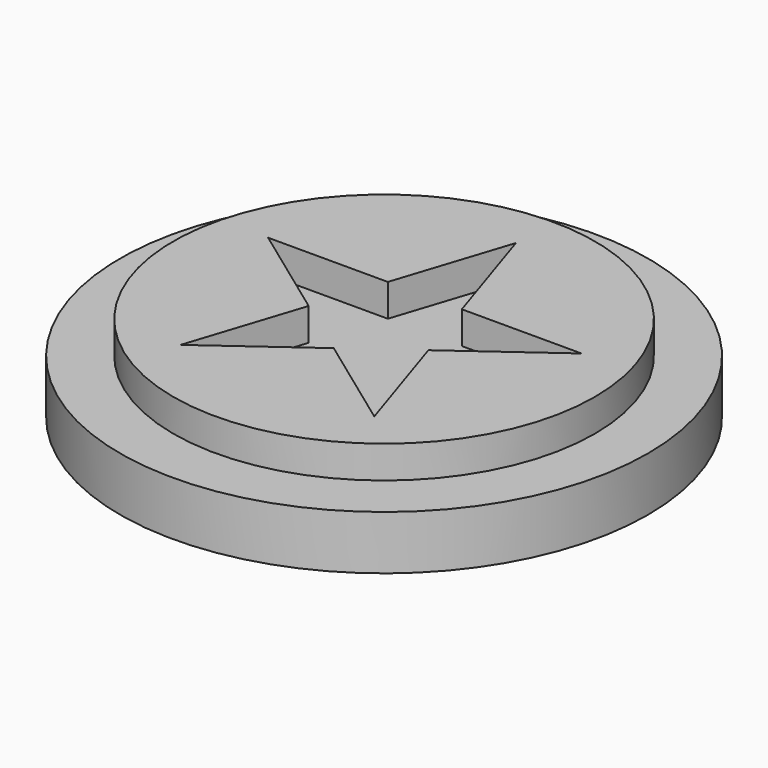
from build123d import *

# Parameters (mm, degrees)
F0_R     = 19.5
F1_DEPTH = 3
F2_R     = 24.4231791104
F3_DEPTH = 5


# Not quite as in the source:
# - a feature of the source that left no trace in its solid (it failed there, or was rolled back) is left out


with BuildPart() as f1:
    # F0 (on Top) → F1 (new body)
    with BuildSketch(Plane.XY):
        with Locations((6.52368e-05, -6.45803e-05)):
            Circle(F0_R)
        Polygon((6.52368e-05, -5.823595641), (-8.9614276, -12.3345013014), (-5.5384419263, -1.7996346453), (-14.4999347632, 4.7112710151), (-3.4229204369, 4.7112710151), (6.52368e-05, 15.2461376711), (3.4230509106, 4.7112710151), (14.5000652368, 4.7112710151), (5.5385724, -1.7996346453), (8.9615580737, -12.3345013014), align=None, mode=Mode.SUBTRACT)
    extrude(amount=F1_DEPTH)


with BuildPart() as f3:
    # F2 (on face) → F3 (new body)
    with BuildSketch(Plane(origin=(0, 0, 0), x_dir=(1, 0, 0), z_dir=(0, 0, -1))):
        with Locations((6.52368e-05, 6.45803e-05)):
            Circle(F2_R)
    extrude(amount=F3_DEPTH)


solid = Compound([f1.part, f3.part])
